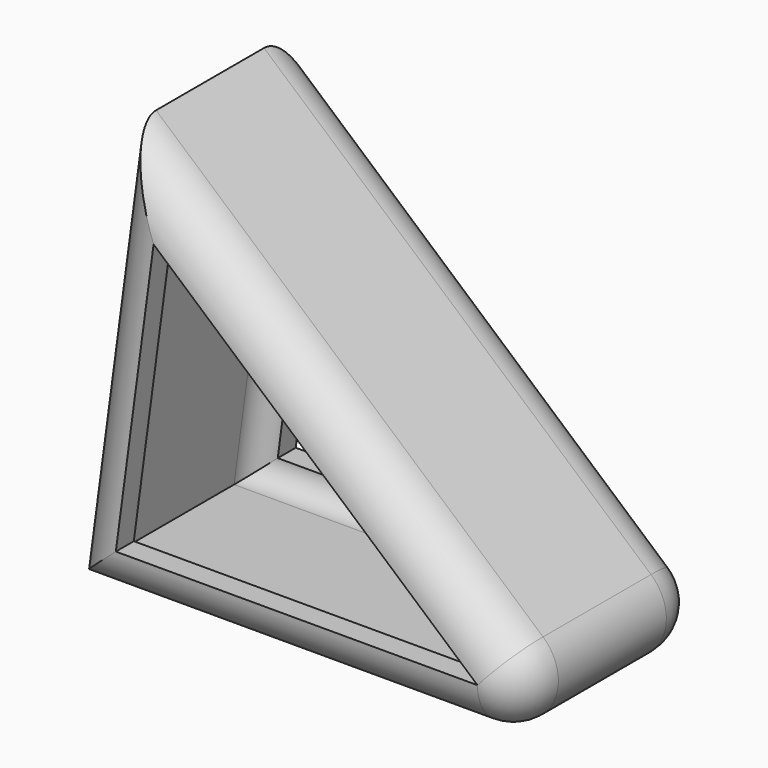
from build123d import *

# Parameters (mm, degrees)
F1_DEPTH = 25.4
F2_R     = 5.08
F3_T     = -2.54


# Not quite as in the source:
# - a shell that OpenCascade refuses in one call is made with other operations: the cavity is built on its own and cut out


with BuildPart() as f1:
    # F0 (on Front) → F1 (new body)
    with BuildSketch(Plane.XZ):
        Polygon((35.6235019863, 0), (-18.2880014181, 47.0535010099), (-24.5744995773, 0), align=None)
    extrude(amount=F1_DEPTH)

    # F2
    f2_edges = [f1.edges().sort_by_distance(p)[0] for p in [
        (8.66775, -25.4, 23.526751),
        (-21.43125, -25.4, 23.526751),
        (5.524501, -25.4, 0),
        (35.623502, -12.7, 0),
        (8.66775, 0, 23.526751),
        (-21.43125, 0, 23.526751),
        (5.524501, 0, 0),
    ]]
    fillet(f2_edges, radius=F2_R)

    # F3: a shell. OpenCascade refuses it in one call, so the cavity is built on its own and cut out:
    # the body offset inwards by the wall thickness, plus a prism from it out through each open face.
    f3_core = offset(f1.part, amount=F3_T, mode=Mode.PRIVATE)
    f3_exits = [f3_core.faces().sort_by_distance(p)[0] for p in [
        (-3.732644, -2.54, 15.722949),
        (-3.732644, -22.86, 15.722949),
    ]]
    add(f3_core, mode=Mode.SUBTRACT)
    extrude(f3_exits, amount=-F3_T, mode=Mode.SUBTRACT)


solid = f1.part
